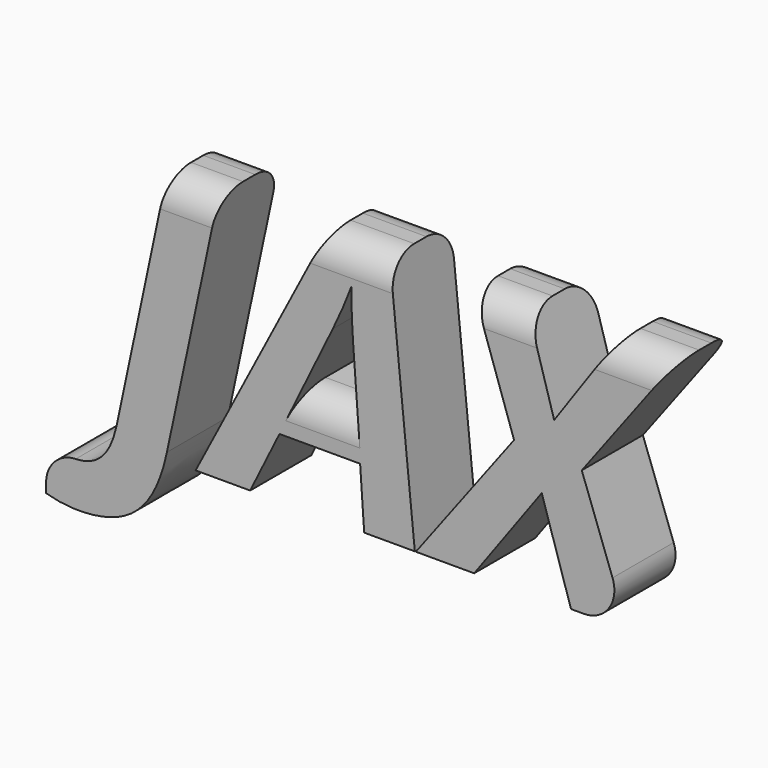
from build123d import *

# Parameters (mm, degrees)
F0_TEXT_SIZE = 58.0319462137
F1_DEPTH     = 12.7
F2_R         = 5.08
F3_SCALE     = 2


# Not quite as in the source:
# - Text() gives the source's letters only with a copy of the font that has no kerning and outlines rounded to 1/6400 em; it was checked with that copy


with BuildPart() as f1:
    # F0 (on Front) → F1 (new body)
    with BuildSketch(Plane.XZ):
        with Locations((-70.6754997373, -21.7805001885)):
            Text('JAX', F0_TEXT_SIZE, font='Open Sans', font_style=FontStyle.BOLDITALIC, text_align=(TextAlign.LEFT, TextAlign.BOTTOM))
    extrude(amount=F1_DEPTH)

    # F2
    f2_edges = [f1.edges().sort_by_distance(p)[0] for p in [
        (-55.446648, -12.7, 19.648869),
        (-27.958547, -12.7, 19.821151),
        (-4.219854, -12.7, 19.648869),
        (19.804465, -12.7, 19.648869),
        (19.804465, 0, 19.648869),
        (-4.219854, 0, 19.648869),
        (-27.958547, 0, 19.821151),
        (-55.446648, 0, 19.648869),
        (-79.797396, -6.35, -26.033154),
        (-32.746182, -12.7, -4.552266),
        (16.834862, -6.35, -21.7805),
    ]]
    fillet(f2_edges, radius=F2_R)


with BuildPart() as f1_1:
    # F3: moved
    add(f1.part.scale(F3_SCALE))


solid = f1_1.part
